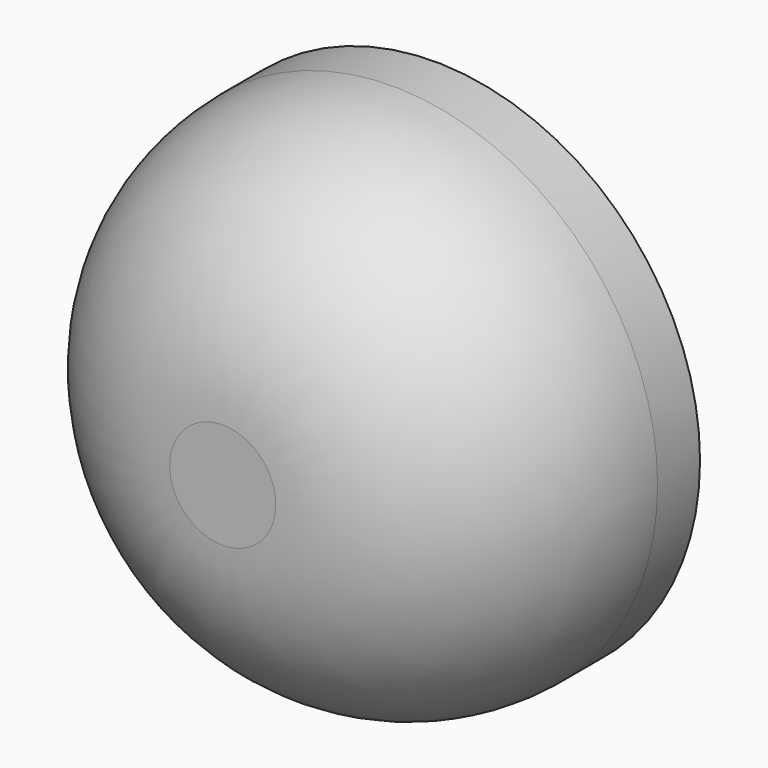
from build123d import *

# Parameters (mm, degrees)
F0_R     = 127
F1_DEPTH = 127
F2_R     = 101.6


# Not quite as in the source:
# - the program builds the solid bodies; features that only make, move or delete a surface that nothing else refers to are left out


with BuildPart() as f1:
    # F0 (on Front) → F1 (new body)
    with BuildSketch(Plane.XZ):
        Circle(F0_R)
    extrude(amount=F1_DEPTH)

    # F2
    f2_edges = [f1.edges().sort_by_distance(p)[0] for p in [
        (-127, -127, 0),
    ]]
    fillet(f2_edges, radius=F2_R)


solid = f1.part
